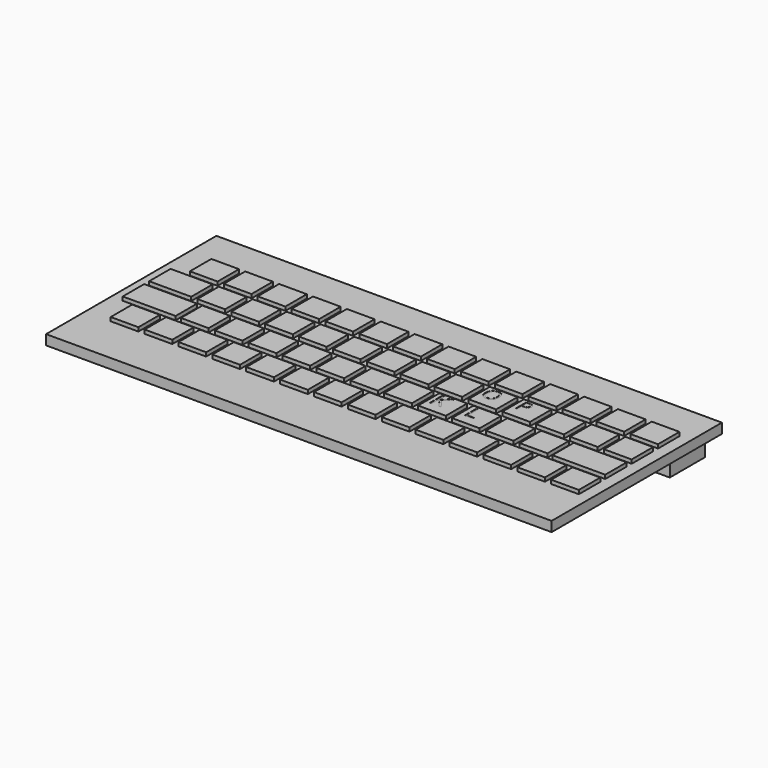
from build123d import *

# Parameters (mm, degrees)
F0_W          = 285
F0_H          = 120
F1_DEPTH      = 5.6
F2_W          = 15.6
F2_H          = 15.1
F2_W_2        = 23.7
F2_W_3        = 29.8
F3_DEPTH      = 2.15
F4_TEXT_SIZE  = 10.3050752336
F5_DEPTH      = 0.1
F6_TEXT_SIZE  = 11.3674969826
F7_DEPTH      = 0.1
F8_TEXT_SIZE  = 12.1084533425
F9_DEPTH      = 0.1
F10_TEXT_SIZE = 12.3491614229
F11_DEPTH     = 0.1
F13_W         = 269.4
F13_H         = 25
F14_DEPTH     = 13.25


# Not quite as in the source:
# - Text() gives the source's letters only with a copy of the font that has no kerning and outlines rounded to 1/6400 em; it was checked with that copy


with BuildPart() as f1:
    # F0 (on Top) → F1 (new body)
    with BuildSketch(Plane.XY):
        Rectangle(F0_W, F0_H)
    extrude(amount=-F1_DEPTH)

    # F2 (on face) → F3 (join)
    with BuildSketch(Plane.XY):
        with Locations((-120.1, 30.65)):
            Rectangle(F2_W, F2_H)
        with Locations((-124.15, 12.0499998063)):
            Rectangle(F2_W_2, F2_H)
        with Locations((-121.1, -6.55)):
            Rectangle(F2_W_3, F2_H)
        with Locations((-101, 12.05)):
            Rectangle(F2_W, F2_H)
        with Locations((-101, 30.65)):
            Rectangle(F2_W, F2_H)
        with Locations((-38.1000119686, -6.5500002623)):
            Rectangle(F2_W, F2_H)
        with Locations((38.2999880314, -6.5500002623)):
            Rectangle(F2_W, F2_H)
        with Locations((57.3999880314, -6.5500002623)):
            Rectangle(F2_W, F2_H)
        with Locations((32.7, 12.05)):
            Rectangle(F2_W, F2_H)
        with Locations((-24.6, -25.15)):
            Rectangle(F2_W, F2_H)
        with Locations((51.8, -25.15)):
            Rectangle(F2_W, F2_H)
        with Locations((51.8, 30.65)):
            Rectangle(F2_W, F2_H)
        with Locations((76.4999880314, -6.5500002623)):
            Rectangle(F2_W, F2_H)
        with Locations((-81.9, 30.65)):
            Rectangle(F2_W, F2_H)
        with Locations((70.9, -25.15)):
            Rectangle(F2_W, F2_H)
        with Locations((128.2, 30.65)):
            Rectangle(F2_W, F2_H)
        with Locations((128.2, 12.05)):
            Rectangle(F2_W, F2_H)
        with Locations((-5.5, 30.65)):
            Rectangle(F2_W, F2_H)
        with Locations((121.1, -6.5500002623)):
            Rectangle(F2_W_3, F2_H)
        with Locations((128.2, -25.15)):
            Rectangle(F2_W, F2_H)
        with Locations((109.1, 30.65)):
            Rectangle(F2_W, F2_H)
        with Locations((109.1, 12.05)):
            Rectangle(F2_W, F2_H)
        with Locations((-5.5, -25.15)):
            Rectangle(F2_W, F2_H)
        with Locations((-81.9, -25.15)):
            Rectangle(F2_W, F2_H)
        with Locations((-19.0000119686, -6.5500002623)):
            Rectangle(F2_W, F2_H)
        with Locations((-62.8, 30.65)):
            Rectangle(F2_W, F2_H)
        with Locations((13.6, 30.65)):
            Rectangle(F2_W, F2_H)
        with Locations((19.1999880314, -6.5500002623)):
            Rectangle(F2_W, F2_H)
        with Locations((-43.7, 30.65)):
            Rectangle(F2_W, F2_H)
        with Locations((90, -25.15)):
            Rectangle(F2_W, F2_H)
        with Locations((70.9, 30.65)):
            Rectangle(F2_W, F2_H)
        with Locations((95.5999880314, -6.5500002623)):
            Rectangle(F2_W, F2_H)
        with Locations((90, 30.65)):
            Rectangle(F2_W, F2_H)
        with Locations((109.1, -25.15)):
            Rectangle(F2_W, F2_H)
        with Locations((13.6, -25.15)):
            Rectangle(F2_W, F2_H)
        with Locations((-62.8, -25.15)):
            Rectangle(F2_W, F2_H)
        with Locations((-43.7, -25.15)):
            Rectangle(F2_W, F2_H)
        with Locations((32.7, -25.15)):
            Rectangle(F2_W, F2_H)
        with Locations((51.8, 12.05)):
            Rectangle(F2_W, F2_H)
        with Locations((-24.6, 12.05)):
            Rectangle(F2_W, F2_H)
        with Locations((-43.7, 12.05)):
            Rectangle(F2_W, F2_H)
        with Locations((-62.8, 12.05)):
            Rectangle(F2_W, F2_H)
        with Locations((13.6, 12.05)):
            Rectangle(F2_W, F2_H)
        with Locations((-24.6, 30.65)):
            Rectangle(F2_W, F2_H)
        with Locations((-57.2000119686, -6.5500002623)):
            Rectangle(F2_W, F2_H)
        with Locations((-5.5, 12.05)):
            Rectangle(F2_W, F2_H)
        with Locations((-81.9, 12.05)):
            Rectangle(F2_W, F2_H)
        with Locations((32.7, 30.65)):
            Rectangle(F2_W, F2_H)
        with Locations((70.9, 12.05)):
            Rectangle(F2_W, F2_H)
        with Locations((-76.3000119686, -6.5500002623)):
            Rectangle(F2_W, F2_H)
        with Locations((90, 12.05)):
            Rectangle(F2_W, F2_H)
        with Locations((0.0999880314, -6.5500002623)):
            Rectangle(F2_W, F2_H)
        with Locations((-95.4000119686, -6.5500002623)):
            Rectangle(F2_W, F2_H)
        with Locations((-101, -25.15)):
            Rectangle(F2_W, F2_H)
        with Locations((-120.1, -25.15)):
            Rectangle(F2_W, F2_H)
    extrude(amount=F3_DEPTH)

    # F4 (on face) → F5 (cut)
    with BuildSketch(Plane.XY.offset(2.15)):
        with Locations((64.7845044732, 10.6858508661)):
            Text('P', F4_TEXT_SIZE, font='Open Sans', text_align=(TextAlign.LEFT, TextAlign.BOTTOM))
    extrude(amount=-F5_DEPTH, mode=Mode.SUBTRACT)

    # F6 (on face) → F7 (cut)
    with BuildSketch(Plane.XY.offset(2.15)):
        with Locations((45.3218556941, 10.0217452273)):
            Text('O', F6_TEXT_SIZE, font='Open Sans', text_align=(TextAlign.LEFT, TextAlign.BOTTOM))
    extrude(amount=-F7_DEPTH, mode=Mode.SUBTRACT)

    # F8 (on face) → F9 (cut)
    with BuildSketch(Plane.XY.offset(2.15)):
        with Locations((51.2271821499, -8.7180864066)):
            Text('L', F8_TEXT_SIZE, font='Open Sans', text_align=(TextAlign.LEFT, TextAlign.BOTTOM))
    extrude(amount=-F9_DEPTH, mode=Mode.SUBTRACT)

    # F10 (on face) → F11 (cut)
    with BuildSketch(Plane.XY.offset(2.15)):
        with Locations((31.7298024893, -8.8913962245)):
            Text('K', F10_TEXT_SIZE, font='Open Sans', text_align=(TextAlign.LEFT, TextAlign.BOTTOM))
    extrude(amount=-F11_DEPTH, mode=Mode.SUBTRACT)

    # F13 (on face) → F14 (join)
    with BuildSketch(Plane(origin=(0, 0, -5.6), x_dir=(1, 0, 0), z_dir=(0, 0, -1))):
        with Locations((0, -45.4999983311)):
            Rectangle(F13_W, F13_H)
    extrude(amount=F14_DEPTH)


solid = f1.part
